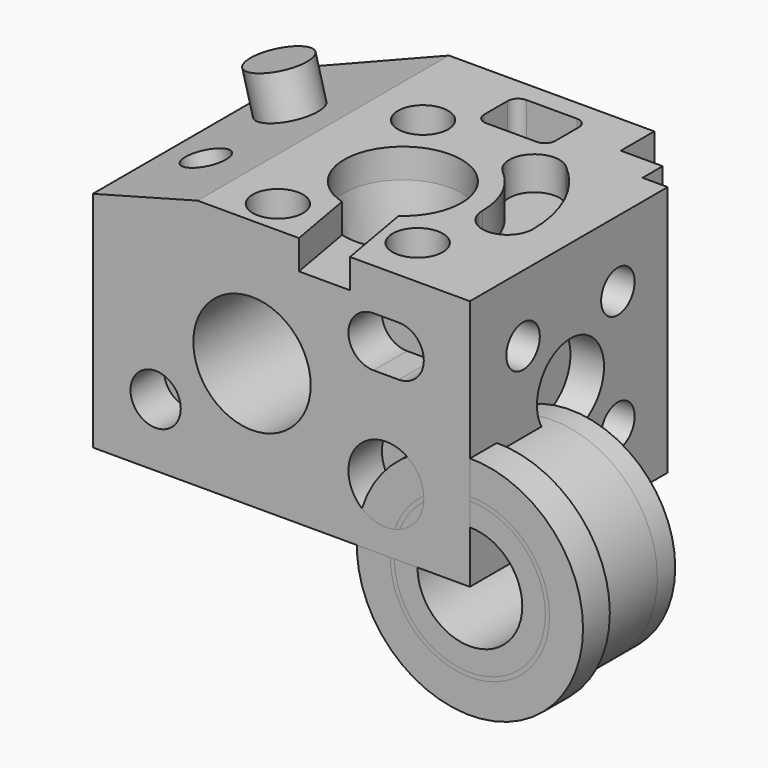
from build123d import *

# Parameters (mm, degrees)
F6_W      = 90
F6_H      = 75
F7_DEPTH  = 60
F9_DEPTH  = 75.001
F11_DEPTH = 87.001
F15_R     = 6.5
F16_DEPTH = 33.1655091949
F17_R     = 6
F18_DEPTH = 8
F20_DEPTH = 7
F22_DEPTH = 60.001
F24_DEPTH = 8
F26_DEPTH = 10
F28_DEPTH = 8
F29_R     = 9
F30_DEPTH = 10
F31_R     = 14
F31_R_2   = 6
F32_DEPTH = 30
F33_DEPTH = 75.001
F34_R     = 6
F35_DEPTH = 10
F36_R     = 10
F36_R_2   = 3
F37_DEPTH = 8
F38_R     = 10
F38_R_2   = 5
F39_DEPTH = 8
F40_R     = 5
F41_DEPTH = 12
F40_R_2   = 7
F42_DEPTH = 10
F43_DEPTH = 10


with BuildPart() as f1:
    # F0 (on Top) → F1 (revolve)
    with BuildSketch(Plane.XY):
        Polygon((12.5, 0), (14.1446864875, 0), (25, 0), (25, 30), (21, 30), (21, 29.6), (19, 29.6), (19, 10), (12.5, 10), align=None)
    revolve(axis=Axis((0, 18.6632340774, 0), (0, -1, 0)))


with BuildPart() as f3:
    # F2 (on Top) → F3 (revolve)
    with BuildSketch(Plane.XY):
        Polygon((19, 0), (27, 0), (27, 8), (25, 8), (25, 24.6872753246), (20, 24.6), (20, 25), (19, 25), align=None)
    revolve(axis=Axis((0, 13.7950675562, 0), (0, -1, 0)))


with BuildPart() as f5:
    # F4 (on Top) → F5 (revolve)
    with BuildSketch(Plane.XY):
        Polygon((12.5, 26), (12.5, 0), (18, 0), (18, 7.6), (16, 7.6), (16, 28.0777988925), (14.35, 28.0777988925), (14.2, 28.9777988925), (11.55, 29), (11.2, 28.5828862426), (11.2, 26), align=None)
    revolve(axis=Axis((0, 15.8516195952, 0), (0, -1, 0)))


with BuildPart() as f7:
    # F6 (on Top) → F7 (new body)
    with BuildSketch(Plane.XY):
        with Locations((-45, 37.5)):
            Rectangle(F6_W, F6_H)
    extrude(amount=F7_DEPTH)

    # F8 (on face) → F9 (cut, through all)
    with BuildSketch(Plane.XZ):
        Polygon((-90, 60), (-90, 53.3012701892), (-65, 60), align=None)
    extrude(amount=-F9_DEPTH, mode=Mode.SUBTRACT)

    # F10 (on face) → F11 (cut, through all)
    with BuildSketch(Plane.XY.offset(60)):
        Polygon((0, 75), (-16, 75), (-16, 65), (-6, 65), (-6, 59), (0, 59), align=None)
    extrude(amount=-F11_DEPTH, mode=Mode.SUBTRACT)

    # F13 (on offset) → F14 (revolve, cut)
    with BuildSketch(Plane.XZ.offset(-30)):
        Polygon((-26, 53), (-26, 60), (-40, 60), (-40, 6.1645091949), (-29, 6.1645091949), (-29, 30.2127376618), align=None)
    revolve(axis=Axis((-40, 30, 33.0822545975), (0, 0, 1)), mode=Mode.SUBTRACT)

    # F15 (on face) → F16 (cut, through all)
    with BuildSketch(Plane.XY.offset(6.1645091949)):
        with Locations((-40, 30)):
            Circle(F15_R)
    extrude(amount=-F16_DEPTH, mode=Mode.SUBTRACT)

    # F17 (on face) → F18 (cut)
    with BuildSketch(Plane.XY.offset(60)):
        with Locations((-52.5, 51.6506350946)):
            Circle(F17_R)
        with Locations((-52.5, 8.3493649054)):
            Circle(F17_R)
        with Locations((-22.3223304703, 12.3223304703)):
            Circle(F17_R)
    extrude(amount=-F18_DEPTH, mode=Mode.SUBTRACT)

    # F19 (on face) → F20 (cut)
    with BuildSketch(Plane.XY.offset(60)):
        with BuildLine():
            ThreePointArc((-31.8946584701, 18.5849468384), (-37.5689255127, 16.2126914578), (-43.7123515062, 16.5011687064))
            Line((-43.7123515062, 16.5011687064), (-40.8027502501, 0))
            Line((-40.8027502501, 0), (-28.6176309074, 0))
            Line((-28.6176309074, 0), (-31.8946584701, 18.5849468384))
        make_face()
    extrude(amount=-F20_DEPTH, mode=Mode.SUBTRACT)

    # F21 (on face) → F22 (cut, through all)
    with BuildSketch(Plane(origin=(0, 0, 0), x_dir=(1, 0, 0), z_dir=(0, 0, -1))):
        Polygon((-65, -75), (-90, -65.9007441433), (-90, -75), align=None)
    extrude(amount=-F22_DEPTH, mode=Mode.SUBTRACT)

    # F23 (on face) → F24 (cut)
    with BuildSketch(Plane.XY.offset(60)):
        with BuildLine():
            Line((-42.5, 58), (-30.5, 58))
            ThreePointArc((-30.5, 58), (-28.732233047, 58.732233047), (-28, 60.5))
            Line((-28, 60.5), (-28, 67.5))
            ThreePointArc((-28, 67.5), (-28.732233047, 69.267766953), (-30.5, 70))
            Line((-30.5, 70), (-42.5, 70))
            ThreePointArc((-42.5, 70), (-44.267766953, 69.267766953), (-45, 67.5))
            Line((-45, 67.5), (-45, 60.5))
            ThreePointArc((-45, 60.5), (-44.267766953, 58.732233047), (-42.5, 58))
        make_face()
    extrude(amount=-F24_DEPTH, mode=Mode.SUBTRACT)

    # F25 (on face) → F26 (cut)
    with BuildSketch(Plane.XZ):
        with BuildLine():
            Line((-23, 38), (-17, 38))
            ThreePointArc((-17, 38), (-11, 44), (-17, 50))
            Line((-17, 50), (-23, 50))
            ThreePointArc((-23, 50), (-29, 44), (-23, 38))
        make_face()
    extrude(amount=-F26_DEPTH, mode=Mode.SUBTRACT)

    # F27 (on face) → F28 (cut)
    with BuildSketch(Plane.XY.offset(60)):
        with BuildLine():
            ThreePointArc((-27.787035416, 44.5548444193), (-22.7801520463, 38.0297469731), (-21, 30))
            ThreePointArc((-21, 30), (-15, 24), (-9, 30))
            ThreePointArc((-9, 30), (-11.9044586019, 43.101166114), (-20.0735840997, 53.7473777367))
            ThreePointArc((-20.0735840997, 53.7473777367), (-28.5265764166, 53.0078367361), (-27.787035416, 44.5548444193))
        make_face()
    extrude(amount=-F28_DEPTH, mode=Mode.SUBTRACT)

    # F29 (on face) → F30 (cut)
    with BuildSketch(Plane.XZ):
        with Locations((-20, 15)):
            Circle(F29_R)
    extrude(amount=-F30_DEPTH, mode=Mode.SUBTRACT)

    # F31 (on face) → F32 (cut)
    with BuildSketch(Plane.XZ):
        with Locations((-52, 30)):
            Circle(F31_R)
        with Locations((-52, 30)):
            Circle(F31_R_2, mode=Mode.SUBTRACT)
    extrude(amount=-F32_DEPTH, mode=Mode.SUBTRACT)

    # F33 (cut, through all): a face of the model
    f33_faces = [f7.faces().sort_by_distance(p)[0] for p in [
        (-52, 0, 30),
    ]]
    extrude(f33_faces, amount=-F33_DEPTH, mode=Mode.SUBTRACT)

    # F34 (on face) → F35 (cut)
    with BuildSketch(Plane.XZ):
        with Locations((-75, 15)):
            Circle(F34_R)
    extrude(amount=-F35_DEPTH, mode=Mode.SUBTRACT)

    # F36 (on face) → F37 (cut)
    with BuildSketch(Plane(origin=(-90, 0, 0), x_dir=(0, -1, 0), z_dir=(-1, 0, 0))):
        with Locations((-30, 30)):
            Circle(F36_R)
        with Locations((-30, 30)):
            Circle(F36_R_2, mode=Mode.SUBTRACT)
    extrude(amount=-F37_DEPTH, mode=Mode.SUBTRACT)

    # F38 (on face) → F39 (cut)
    with BuildSketch(Plane.YZ):
        with Locations((30, 30)):
            Circle(F38_R)
        with Locations((15.8578643763, 44.1421356237)):
            Circle(F38_R_2)
        with Locations((44.1421356237, 44.1421356237)):
            Circle(F38_R_2)
        with Locations((44.1421356237, 15.8578643763)):
            Circle(F38_R_2)
        with Locations((15.8578643763, 15.8578643763)):
            Circle(F38_R_2)
    extrude(amount=-F39_DEPTH, mode=Mode.SUBTRACT)

    # F40 (on face) → F41 (cut)
    with BuildSketch(Plane(origin=(-19.354174377, 0, 72.2307621135), x_dir=(0.9659258263, 0, 0.2588190451), z_dir=(-0.2588190451, 0, 0.9659258263))):
        with Locations((-61.7499405129, 45)):
            Circle(F40_R)
        with Locations((-61.7499405129, 20)):
            Circle(F40_R)
    extrude(amount=-F41_DEPTH, mode=Mode.SUBTRACT)

    # F40 (on face) → F42 (join)
    with BuildSketch(Plane(origin=(-19.354174377, 0, 72.2307621135), x_dir=(0.9659258263, 0, 0.2588190451), z_dir=(-0.2588190451, 0, 0.9659258263))):
        with Locations((-61.7499405129, 45)):
            Circle(F40_R_2)
        with Locations((-61.7499405129, 45)):
            Circle(F40_R, mode=Mode.SUBTRACT)
    extrude(amount=F42_DEPTH)

    # F40 (on face) → F43 (join)
    with BuildSketch(Plane(origin=(-19.354174377, 0, 72.2307621135), x_dir=(0.9659258263, 0, 0.2588190451), z_dir=(-0.2588190451, 0, 0.9659258263))):
        with Locations((-61.7499405129, 45)):
            Circle(F40_R)
    extrude(amount=F43_DEPTH)


solid = Compound([f1.part, f3.part, f5.part, f7.part])
